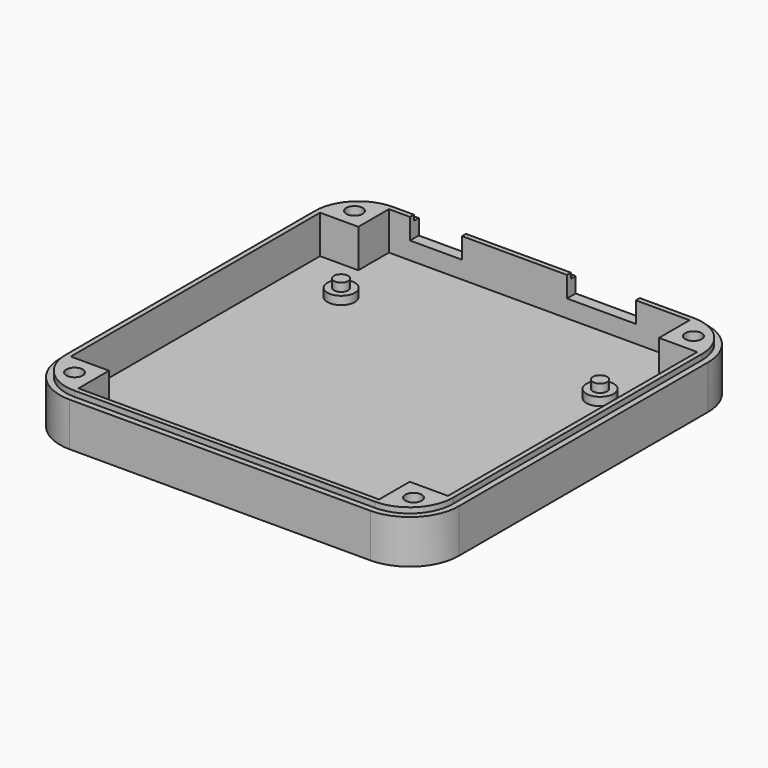
from build123d import *

# Parameters (mm, degrees)
F1_DEPTH  = 2
F2_R      = 2.5
F3_DEPTH  = 1.5
F4_R      = 1.3
F5_DEPTH  = 1.5
F7_DEPTH  = 7
F8_R      = 1.5
F9_DEPTH  = 10
F10_W     = 12.6
F10_H     = 2
F10_W_2   = 9.5
F11_DEPTH = 3.8
F12_R     = 3
F13_DEPTH = 0.4
F14_SIZE  = 1.49999
F15_W     = 19.2
F15_H     = 1.1
F16_DEPTH = 1


# Not quite as in the source:
# - a fillet or chamfer is up to 0.001 mm smaller than in the source, because OpenCascade refuses the exact size


with BuildPart() as f1:
    # F0 (on Top) → F1 (new body)
    with BuildSketch(Plane.XY):
        with BuildLine():
            Line((27.5, 38.5), (-27.5, 38.5))
            ThreePointArc((-27.5, 38.5), (-33.8639610307, 35.8639610307), (-36.5, 29.5))
            Line((-36.5, 29.5), (-36.5, -27.5))
            ThreePointArc((-36.5, -27.5), (-33.8639610307, -33.8639610307), (-27.5, -36.5))
            Line((-27.5, -36.5), (27.5, -36.5))
            ThreePointArc((27.5, -36.5), (33.8639610307, -33.8639610307), (36.5, -27.5))
            Line((36.5, -27.5), (36.5, 29.5))
            ThreePointArc((36.5, 29.5), (33.8639610307, 35.8639610307), (27.5, 38.5))
        make_face()
    extrude(amount=F1_DEPTH)

    # F2 (on face) → F3 (join)
    with BuildSketch(Plane.XY.offset(2)):
        with Locations((-19.24, -30.6)):
            Circle(F2_R)
        with Locations((8.96, -30.6)):
            Circle(F2_R)
        with Locations((24.16, 20.2)):
            Circle(F2_R)
        with Locations((-24.24, 21.5)):
            Circle(F2_R)
    extrude(amount=F3_DEPTH)

    # F4 (on face) → F5 (join)
    with BuildSketch(Plane.XY.offset(3.5)):
        with Locations((-19.24, -30.6)):
            Circle(F4_R)
        with Locations((8.96, -30.6)):
            Circle(F4_R)
        with Locations((24.16, 20.2)):
            Circle(F4_R)
        with Locations((-24.24, 21.5)):
            Circle(F4_R)
    extrude(amount=F5_DEPTH)

    # F6 (on face) → F7 (join)
    with BuildSketch(Plane.XY.offset(2)):
        with BuildLine():
            Line((27.5, 38.5), (-27.5, 38.5))
            ThreePointArc((-27.5, 38.5), (-33.8639610307, 35.8639610307), (-36.5, 29.5))
            Line((-36.5, 29.5), (-36.5, -27.5))
            ThreePointArc((-36.5, -27.5), (-33.8639610307, -33.8639610307), (-27.5, -36.5))
            Line((-27.5, -36.5), (27.5, -36.5))
            ThreePointArc((27.5, -36.5), (33.8639610307, -33.8639610307), (36.5, -27.5))
            Line((36.5, -27.5), (36.5, 29.5))
            ThreePointArc((36.5, 29.5), (33.8639610307, 35.8639610307), (27.5, 38.5))
        make_face()
        Polygon((-27.5, 29.5), (-27.5, 36.5), (27.5, 36.5), (27.5, 29.5), (34.5, 29.5), (34.5, -27.5), (27.5, -27.5), (27.5, -34.5), (-27.5, -34.5), (-27.5, -27.5), (-34.5, -27.5), (-34.5, 29.5), align=None, mode=Mode.SUBTRACT)
    extrude(amount=F7_DEPTH)

    # F8 (on face) → F9 (cut)
    with BuildSketch(Plane.XY.offset(9)):
        with Locations((-31, 33)):
            Circle(F8_R)
        with Locations((31, 33)):
            Circle(F8_R)
        with Locations((-31, -31)):
            Circle(F8_R)
        with Locations((31, -31)):
            Circle(F8_R)
    extrude(amount=-F9_DEPTH, mode=Mode.SUBTRACT)

    # F10 (on face) → F11 (cut)
    with BuildSketch(Plane.XY.offset(9)):
        with Locations((11.36, 37.5)):
            Rectangle(F10_W, F10_H)
        with Locations((-18.89, 37.5)):
            Rectangle(F10_W_2, F10_H)
    extrude(amount=-F11_DEPTH, mode=Mode.SUBTRACT)

    # F12 (on face) → F13 (cut)
    with BuildSketch(Plane(origin=(0, 0, 0), x_dir=(1, 0, 0), z_dir=(0, 0, -1))):
        with Locations((31, -33)):
            Circle(F12_R)
        with Locations((-31, -33)):
            Circle(F12_R)
        with Locations((-31, 31)):
            Circle(F12_R)
        with Locations((31, 31)):
            Circle(F12_R)
    extrude(amount=-F13_DEPTH, mode=Mode.SUBTRACT)

    # F14 (size 1.5 in the source; OpenCascade refuses exactly that, so slightly less here)
    f14_edges = [f1.edges().sort_by_distance(p)[0] for p in [
        (29.5, 33, 0.4),
        (-32.5, 33, 0.4),
        (29.5, -31, 0.4),
        (-32.5, -31, 0.4),
    ]]
    chamfer(f14_edges, length=F14_SIZE)

    # F15 (on face) → F16 (cut)
    with BuildSketch(Plane.XY.offset(9)):
        with BuildLine():
            Line((-23.64, 38.5), (-27.5, 38.5))
            ThreePointArc((-27.5, 38.5), (-33.8639610307, 35.8639610307), (-36.5, 29.5))
            Line((-36.5, 29.5), (-36.5, -27.5))
            ThreePointArc((-36.5, -27.5), (-33.8639610307, -33.8639610307), (-27.5, -36.5))
            Line((-27.5, -36.5), (27.5, -36.5))
            ThreePointArc((27.5, -36.5), (33.8639610307, -33.8639610307), (36.5, -27.5))
            Line((36.5, -27.5), (36.5, 29.5))
            ThreePointArc((36.5, 29.5), (33.8639610307, 35.8639610307), (27.5, 38.5))
            Line((27.5, 38.5), (17.66, 38.5))
            Line((17.66, 38.5), (17.66, 37.4))
            Line((17.66, 37.4), (27.5, 37.4))
            ThreePointArc((27.5, 37.4), (33.0861435714, 35.0861435714), (35.4, 29.5))
            Line((35.4, 29.5), (35.4, -27.5))
            ThreePointArc((35.4, -27.5), (33.0861435714, -33.0861435714), (27.5, -35.4))
            Line((27.5, -35.4), (-27.5, -35.4))
            ThreePointArc((-27.5, -35.4), (-33.0861435714, -33.0861435714), (-35.4, -27.5))
            Line((-35.4, -27.5), (-35.4, 29.5))
            ThreePointArc((-35.4, 29.5), (-33.0861435714, 35.0861435714), (-27.5, 37.4))
            Line((-27.5, 37.4), (-23.64, 37.4))
            Line((-23.64, 37.4), (-23.64, 38.5))
        make_face()
        with Locations((-4.54, 37.95)):
            Rectangle(F15_W, F15_H)
    extrude(amount=-F16_DEPTH, mode=Mode.SUBTRACT)


solid = f1.part
